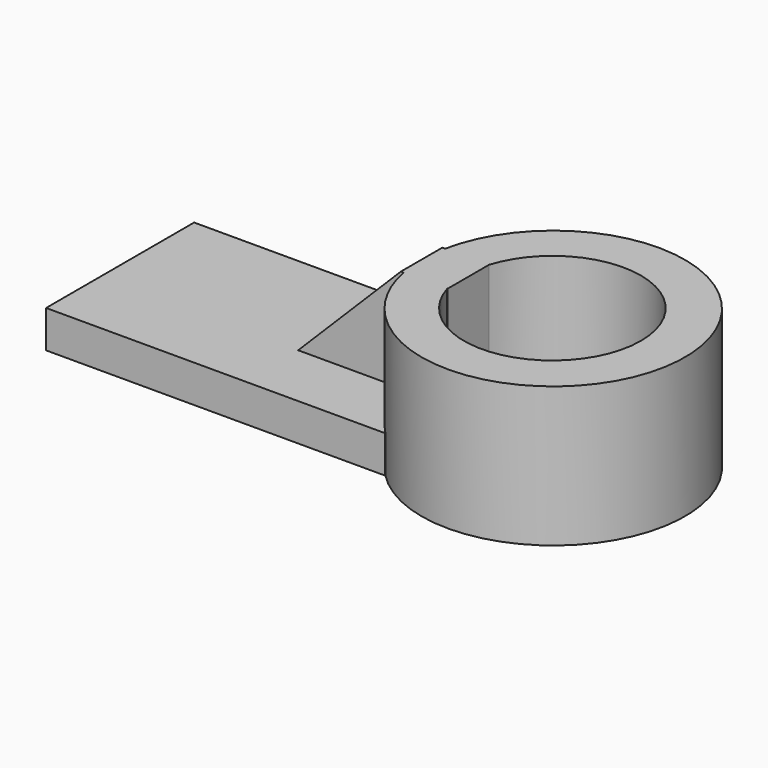
from build123d import *

# Parameters (mm, degrees)
F1_R        = 24.0785224066
F2_DEPTH    = 38.1
F3_DEPTH    = 10.16
F4_W        = 72.8784613311
F4_H        = 14.0676931478
F5_DEPTH    = 38.1
F6_DEPTH    = 0.508
F7_T4_DEPTH = 321.0752082512


# Not quite as in the source:
# - a fillet or chamfer that OpenCascade refuses, or shapes differently, is made with other operations: its cross-section is extruded or revolved along the edge and cut away or added


with BuildPart() as f2:
    # F1 (on face) → F2 (new body)
    with BuildSketch(Plane.XY):
        with BuildLine():
            ThreePointArc((21.3381504126, 25.1467317917), (11.0402076987, 0), (21.3381504126, -25.1467317917))
            ThreePointArc((21.3381504126, -25.1467317917), (60.4791188031, -33.1778787511), (82.7444076987, 0))
            ThreePointArc((82.7444076987, 0), (60.4791188031, 33.1778787511), (21.3381504126, 25.1467317917))
        make_face()
        with Locations((46.6475896537, 0)):
            Circle(F1_R, mode=Mode.SUBTRACT)
    extrude(amount=F2_DEPTH)

    # F0 (on Top) → F3 (join)
    with BuildSketch(Plane.XY):
        with BuildLine():
            ThreePointArc((21.3381504126, -25.1467317917), (11.0402076987, 0), (21.3381504126, 25.1467317917))
            Line((21.3381504126, 25.1467317917), (-70.9246173501, 25.1467317917))
            Line((-70.9246173501, 25.1467317917), (-70.9246173501, -25.1914039254))
            Line((-70.9246173501, -25.1914039254), (21.3381504126, -25.1914039254))
            Line((21.3381504126, -25.1914039254), (21.3381504126, -25.1467317917))
        make_face()
    extrude(amount=F3_DEPTH)

    # F4 (on Top) → F5 (join)
    with BuildSketch(Plane.XY):
        with Locations((-12.2608747333, 0.0976922456)):
            Rectangle(F4_W, F4_H)
    extrude(amount=F5_DEPTH)

    # F6 (cut): a face of the model
    f6_faces = [f2.faces().sort_by_distance(p)[0] for p in [
        (24.1783559322, 0.0976922456, 19.05),
    ]]
    extrude(f6_faces, amount=-F6_DEPTH, mode=Mode.SUBTRACT)

    # F7: chamfer of 59.69 on 1 edges, made by hand


with BuildPart() as f7_tool2:
    # F7_s3 → F7_t4 (new body)
    with BuildSketch(Plane.XZ.offset(-160.6352963712)):
        Polygon((10.9898946011, 38.1), (-48.7001053989, -21.59), (-48.7001053989, 38.1), align=None)
    extrude(amount=F7_T4_DEPTH)

    split(bisect_by=Plane.XY.offset(10.16), keep=Keep.TOP)


with BuildPart() as f2_1:
    add(f2.part)

    # F7_t1: cut F7_tool2
    add(f7_tool2.part, mode=Mode.SUBTRACT)


solid = f2_1.part
